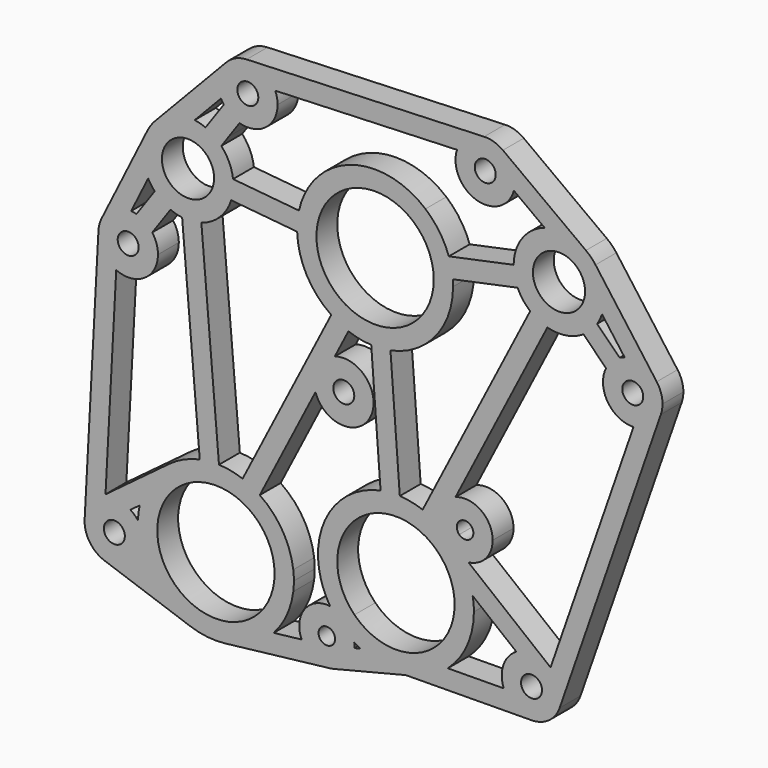
from build123d import *

# Parameters (mm, degrees)
F0_R     = 2.5527
F0_R_2   = 14.2875
F0_R_3   = 6.35
F1_DEPTH = 6.35


# Not quite as in the source:
# - a feature names something its author has since deleted; it is built from what else it names


with BuildPart() as f1:
    # F0 (on Front) → F1 (new body)
    with BuildSketch(Plane.XZ):
        with BuildLine():
            ThreePointArc((10.1027881362, 10.1027881362), (13.1999288208, 5.4675895399), (14.2875, 0))
            ThreePointArc((14.2875, 0), (5.4675895399, -13.1999288208), (-10.1027881362, -10.1027881362))
            Line((-10.1027881362, -10.1027881362), (-12.087424739, -12.087424739))
            ThreePointArc((-12.087424739, -12.087424739), (-10.7962746794, -13.8997241174), (-10.1679167372, -16.0343584679))
            ThreePointArc((-10.1679167372, -16.0343584679), (-9.4333272467, -16.4772424667), (-8.679483979, -16.8864957913))
            ThreePointArc((-8.679483979, -16.8864957913), (-4.3796020882, -18.474476117), (0.1755409055, -18.9856884953))
            ThreePointArc((0.1755409055, -18.9856884953), (2.3991856615, -18.83430621), (4.5897696443, -18.4233872255))
            ThreePointArc((4.5897696443, -18.4233872255), (8.871283082, -16.7865278938), (12.6357418971, -14.1712811333))
            ThreePointArc((12.6357418971, -14.1712811333), (17.326218511, -7.7646206836), (18.9865, 0))
            ThreePointArc((18.9865, 0), (18.9129246484, 1.6698693044), (18.6927688232, 3.3267966532))
            ThreePointArc((18.6927688232, 3.3267966532), (17.6972758772, 6.8770348826), (16.0343584679, 10.1679167372))
            ThreePointArc((16.0343584679, 10.1679167372), (13.8997241174, 10.7962746794), (12.087424739, 12.087424739))
            Line((12.087424739, 12.087424739), (10.1027881362, 10.1027881362))
        make_face()
        with BuildLine():
            ThreePointArc((-10.1027881362, -10.1027881362), (-10.1027881362, 10.1027881362), (10.1027881362, 10.1027881362))
            Line((10.1027881362, 10.1027881362), (12.087424739, 12.087424739))
            ThreePointArc((12.087424739, 12.087424739), (10.7962746794, 13.8997241174), (10.1679167372, 16.0343584679))
            ThreePointArc((10.1679167372, 16.0343584679), (8.3844360103, 17.0349175237), (6.5036895316, 17.8378587484))
            ThreePointArc((6.5036895316, 17.8378587484), (3.7643940626, 18.6095813922), (0.9405215506, 18.9631906984))
            ThreePointArc((0.9405215506, 18.9631906984), (-1.4133229179, 18.933824246), (-3.7454416407, 18.6134050933))
            ThreePointArc((-3.7454416407, 18.6134050933), (-16.2312532017, 9.8505635247), (-18.2403128263, -5.2705))
            Line((-18.2403128263, -5.2705), (-16.1584730714, -5.2705))
            Line((-16.1584730714, -5.2705), (-16.1584730714, -9.9695))
            ThreePointArc((-16.1584730714, -9.9695), (-16.0967214963, -10.0688996082), (-16.0343584679, -10.1679167372))
            ThreePointArc((-16.0343584679, -10.1679167372), (-13.8997241174, -10.7962746794), (-12.087424739, -12.087424739))
            Line((-12.087424739, -12.087424739), (-10.1027881362, -10.1027881362))
        make_face()
        with BuildLine():
            ThreePointArc((10.1679167372, 16.0343584679), (10.7962746794, 13.8997241174), (12.087424739, 12.087424739))
            Line((12.087424739, 12.087424739), (13.425482901, 13.425482901))
            ThreePointArc((13.425482901, 13.425482901), (12.6695294718, 14.1410821797), (11.8754941276, 14.8141763685))
            ThreePointArc((11.8754941276, 14.8141763685), (11.288975975, 15.2658508995), (10.6852962958, 15.6943182496))
            ThreePointArc((10.6852962958, 15.6943182496), (10.4279926298, 15.8664473643), (10.1679167372, 16.0343584679))
        make_face()
        with BuildLine():
            Line((13.425482901, 13.425482901), (12.087424739, 12.087424739))
            ThreePointArc((12.087424739, 12.087424739), (13.8997241174, 10.7962746794), (16.0343584679, 10.1679167372))
            ThreePointArc((16.0343584679, 10.1679167372), (14.8196996494, 11.8686007833), (13.425482901, 13.425482901))
        make_face()
        with BuildLine():
            ThreePointArc((-10.1679167372, -16.0343584679), (-10.7962746794, -13.8997241174), (-12.087424739, -12.087424739))
            Line((-12.087424739, -12.087424739), (-13.425482901, -13.425482901))
            ThreePointArc((-13.425482901, -13.425482901), (-11.8686007833, -14.8196996494), (-10.1679167372, -16.0343584679))
        make_face()
        with BuildLine():
            Line((-13.425482901, -13.425482901), (-12.087424739, -12.087424739))
            ThreePointArc((-12.087424739, -12.087424739), (-13.8997241174, -10.7962746794), (-16.0343584679, -10.1679167372))
            ThreePointArc((-16.0343584679, -10.1679167372), (-14.8196996494, -11.8686007833), (-13.425482901, -13.425482901))
        make_face()
        with BuildLine():
            Line((13.5066179368, 13.5066179368), (13.425482901, 13.425482901))
            ThreePointArc((13.425482901, 13.425482901), (14.8196996494, 11.8686007833), (16.0343584679, 10.1679167372))
            ThreePointArc((16.0343584679, 10.1679167372), (16.8510479224, 10.1196929359), (17.6675435983, 10.1710934346))
            Line((17.6675435983, 10.1710934346), (13.5066179368, 13.5066179368))
        make_face()
        with BuildLine():
            ThreePointArc((11.8754941276, 14.8141763685), (12.6695294718, 14.1410821797), (13.425482901, 13.425482901))
            Line((13.425482901, 13.425482901), (13.5066179368, 13.5066179368))
            Line((13.5066179368, 13.5066179368), (11.8754941276, 14.8141763685))
        make_face()
        with BuildLine():
            ThreePointArc((14.5002054636, 23.1364216251), (11.1025541076, 20.3366145489), (10.1679167372, 16.0343584679))
            ThreePointArc((10.1679167372, 16.0343584679), (10.4279926298, 15.8664473643), (10.6852962958, 15.6943182496))
            Line((10.6852962958, 15.6943182496), (14.5002054636, 23.1364216251))
        make_face()
        with BuildLine():
            ThreePointArc((6.5036895316, 17.8378587484), (8.3844360103, 17.0349175237), (10.1679167372, 16.0343584679))
            ThreePointArc((10.1679167372, 16.0343584679), (11.1025541076, 20.3366145489), (14.5002054636, 23.1364216251))
            Line((14.5002054636, 23.1364216251), (36.8778846589, 66.7906724992))
            ThreePointArc((36.8778846589, 66.7906724992), (34.6718105613, 67.6375732842), (32.6962778947, 68.934212998))
            Line((32.6962778947, 68.934212998), (6.5036895316, 17.8378587484))
        make_face()
        with BuildLine():
            ThreePointArc((17.6675435983, 10.1710934346), (16.8510479224, 10.1196929359), (16.0343584679, 10.1679167372))
            ThreePointArc((16.0343584679, 10.1679167372), (17.6972758772, 6.8770348826), (18.6927688232, 3.3267966532))
            Line((18.6927688232, 3.3267966532), (29.3206645114, -5.1928476183))
            ThreePointArc((29.3206645114, -5.1928476183), (33.5286304822, -4.1961595316), (37.555723844, -5.7718764506))
            Line((37.555723844, -5.7718764506), (17.6675435983, 10.1710934346))
        make_face()
        with BuildLine():
            ThreePointArc((-10.1679167372, -16.0343584679), (-11.8686007833, -14.8196996494), (-13.425482901, -13.425482901))
            ThreePointArc((-13.425482901, -13.425482901), (-14.8196996494, -11.8686007833), (-16.0343584679, -10.1679167372))
            ThreePointArc((-16.0343584679, -10.1679167372), (-22.2468220658, -12.8530103585), (-22.970288636, -19.5821282674))
            ThreePointArc((-22.970288636, -19.5821282674), (-20.1602814757, -22.6773183147), (-16.0638899585, -23.5115354374))
            ThreePointArc((-16.0638899585, -23.5115354374), (-15.6364127746, -23.447956819), (-15.2139078913, -23.3570249376))
            ThreePointArc((-15.2139078913, -23.3570249376), (-11.6731694063, -21.1345234976), (-10.1322290579, -17.2484143236))
            ThreePointArc((-10.1322290579, -17.2484143236), (-10.1228181675, -17.0432931715), (-10.119680227, -16.837980227))
            ThreePointArc((-10.119680227, -16.837980227), (-10.1317501969, -16.4354461624), (-10.1679167372, -16.0343584679))
        make_face()
        with BuildLine():
            ThreePointArc((-14.818680227, -16.837980227), (-18.703570167, -17.610732882), (-15.4101195038, -15.4101195038))
            ThreePointArc((-15.4101195038, -15.4101195038), (-14.972390287, -16.065227572), (-14.818680227, -16.837980227))
        make_face(mode=Mode.SUBTRACT)
        with BuildLine():
            ThreePointArc((10.6852962958, 15.6943182496), (11.288975975, 15.2658508995), (11.8754941276, 14.8141763685))
            Line((11.8754941276, 14.8141763685), (13.5066179368, 13.5066179368))
            Line((13.5066179368, 13.5066179368), (17.6675435983, 10.1710934346))
            ThreePointArc((17.6675435983, 10.1710934346), (21.8732960308, 12.3903797901), (23.556280227, 16.837980227))
            ThreePointArc((23.556280227, 16.837980227), (20.6739731035, 22.3534778058), (14.5002054636, 23.1364216251))
            Line((14.5002054636, 23.1364216251), (10.6852962958, 15.6943182496))
        make_face()
        with BuildLine():
            ThreePointArc((18.857280227, 16.837980227), (17.610732882, 14.972390287), (15.4101195038, 15.4101195038))
            ThreePointArc((15.4101195038, 15.4101195038), (16.065227572, 18.703570167), (18.857280227, 16.837980227))
        make_face(mode=Mode.SUBTRACT)
        with BuildLine():
            ThreePointArc((0.1755409055, -18.9856884953), (-4.3796020882, -18.474476117), (-8.679483979, -16.8864957913))
            Line((-8.679483979, -16.8864957913), (-10.1322290579, -17.2484143236))
            ThreePointArc((-10.1322290579, -17.2484143236), (-11.6731694063, -21.1345234976), (-15.2139078913, -23.3570249376))
            Line((-15.2139078913, -23.3570249376), (2.4158307327, -18.9649748665))
            Line((2.4158307327, -18.9649748665), (0.1755409055, -18.9856884953))
        make_face()
        with BuildLine():
            ThreePointArc((-18.2403128263, -5.2705), (-17.3591263622, -7.6907681145), (-16.1584730714, -9.9695))
            Line((-16.1584730714, -9.9695), (-16.1584730714, -5.2705))
            Line((-16.1584730714, -5.2705), (-18.2403128263, -5.2705))
        make_face()
        with BuildLine():
            ThreePointArc((-16.0638899585, -23.5115354374), (-20.1602814757, -22.6773183147), (-22.970288636, -19.5821282674))
            Line((-22.970288636, -19.5821282674), (-29.7764261148, -20.371597242))
            ThreePointArc((-29.7764261148, -20.371597242), (-35.161229574, -24.5050380312), (-41.6559027226, -26.4800473337))
            Line((-41.6559027226, -26.4800473337), (-16.0638899585, -23.5115354374))
        make_face()
        with BuildLine():
            ThreePointArc((-3.7454416407, 18.6134050933), (-1.4133229179, 18.933824246), (0.9405215506, 18.9631906984))
            Line((0.9405215506, 18.9631906984), (-1.3345583593, 49.4416911273))
            ThreePointArc((-1.3345583593, 49.4416911273), (-3.6666770821, 49.1212719745), (-6.0205215506, 49.0919055222))
            Line((-6.0205215506, 49.0919055222), (-3.7454416407, 18.6134050933))
        make_face()
        with BuildLine():
            ThreePointArc((29.6298751444, 72.9499771349), (30.9304471577, 70.7644612984), (32.6962778947, 68.934212998))
            ThreePointArc((32.6962778947, 68.934212998), (34.6718105613, 67.6375732842), (36.8778846589, 66.7906724992))
            ThreePointArc((36.8778846589, 66.7906724992), (41.4271180616, 66.5549248717), (45.6848221123, 68.1745105325))
            ThreePointArc((45.6848221123, 68.1745105325), (47.5248502349, 69.6571771747), (49.0075168771, 71.4972052973))
            ThreePointArc((49.0075168771, 71.4972052973), (49.6746613221, 72.6923094988), (50.1889265376, 73.9607286137))
            ThreePointArc((50.1889265376, 73.9607286137), (50.617064307, 75.6922004422), (50.7610274096, 77.47))
            ThreePointArc((50.7610274096, 77.47), (50.208206927, 80.9211761095), (48.6050646005, 84.0270031661))
            ThreePointArc((48.6050646005, 84.0270031661), (47.5248502349, 85.2828228253), (46.2690305758, 86.3630371909))
            ThreePointArc((46.2690305758, 86.3630371909), (41.4293864022, 88.3847184614), (36.2027560234, 87.946899128))
            ThreePointArc((36.2027560234, 87.946899128), (32.5255649938, 85.8625656951), (29.9000958465, 82.55))
            ThreePointArc((29.9000958465, 82.55), (28.9861019442, 80.1223430981), (28.6633062214, 77.5484927125))
            ThreePointArc((28.6633062214, 77.5484927125), (28.8993015921, 75.1972568568), (29.6298751444, 72.9499771349))
        make_face()
        with BuildLine():
            ThreePointArc((46.0620274096, 77.47), (36.8722210782, 71.7903873372), (35.9020274096, 82.55))
            ThreePointArc((35.9020274096, 82.55), (42.551833741, 83.1496126628), (46.0620274096, 77.47))
        make_face(mode=Mode.SUBTRACT)
        with BuildLine():
            ThreePointArc((37.555723844, -5.7718764506), (33.5286304822, -4.1961595316), (29.3206645114, -5.1928476183))
            ThreePointArc((29.3206645114, -5.1928476183), (26.1672444912, -9.0578923239), (26.256338269, -14.0453456519))
            ThreePointArc((26.256338269, -14.0453456519), (28.9476060736, -17.4302300454), (33.0870460582, -18.6813900541))
            ThreePointArc((33.0870460582, -18.6813900541), (37.249950733, -17.3202181358), (39.8698682415, -13.8104323061))
            ThreePointArc((39.8698682415, -13.8104323061), (40.170536428, -12.6370549621), (40.2717, -11.43))
            ThreePointArc((40.2717, -11.43), (39.5862059809, -8.352323619), (37.659321687, -5.8565049409))
            ThreePointArc((37.659321687, -5.8565049409), (37.6077179098, -5.8139518102), (37.555723844, -5.7718764506))
        make_face()
        with Locations((33.02, -11.43)):
            Circle(F0_R, mode=Mode.SUBTRACT)
        with BuildLine():
            ThreePointArc((4.5897696443, -18.4233872255), (2.3991856615, -18.83430621), (0.1755409055, -18.9856884953))
            Line((0.1755409055, -18.9856884953), (2.4158307327, -18.9649748665))
            Line((2.4158307327, -18.9649748665), (4.5897696443, -18.4233872255))
        make_face()
        with BuildLine():
            Line((-25.0029803525, -5.2705), (-25.0029803525, -9.9695))
            ThreePointArc((-25.0029803525, -9.9695), (-24.893567057, -8.7970138243), (-24.8570491337, -7.62))
            ThreePointArc((-24.8570491337, -7.62), (-24.893567057, -6.4429861757), (-25.0029803525, -5.2705))
        make_face()
        with BuildLine():
            ThreePointArc((-29.7764261148, -20.371597242), (-26.5872473381, -15.5387897174), (-25.0029803525, -9.9695))
            Line((-25.0029803525, -9.9695), (-25.0029803525, -5.2705))
            ThreePointArc((-25.0029803525, -5.2705), (-27.6442418047, 2.283010871), (-33.1629165809, 8.0774924915))
            ThreePointArc((-33.1629165809, 8.0774924915), (-35.1875075447, 9.2785243811), (-37.3451600732, 10.2197904099))
            ThreePointArc((-37.3451600732, 10.2197904099), (-40.1777850684, 11.0092607494), (-43.0983409674, 11.3518698878))
            ThreePointArc((-43.0983409674, 11.3518698878), (-45.4517582606, 11.298267512), (-47.7804539971, 10.9538515754))
            ThreePointArc((-47.7804539971, 10.9538515754), (-51.6694427495, 9.6786291759), (-55.1947929153, 7.5996073162))
            ThreePointArc((-55.1947929153, 7.5996073162), (-59.8231534442, 2.6337519149), (-62.4088249945, -3.642850963))
            ThreePointArc((-62.4088249945, -3.642850963), (-62.6907023453, -5.3239167985), (-62.8206763208, -7.0234884945))
            ThreePointArc((-62.8206763208, -7.0234884945), (-61.7115198037, -9.1038158537), (-61.3283, -11.43))
            ThreePointArc((-61.3283, -11.43), (-61.4374580323, -12.6834939688), (-61.761645872, -13.8992508732))
            ThreePointArc((-61.761645872, -13.8992508732), (-61.1262796106, -15.4809420245), (-60.3516188327, -16.9992759349))
            ThreePointArc((-60.3516188327, -16.9992759349), (-55.997100169, -22.2069249495), (-50.088980786, -25.5499125967))
            ThreePointArc((-50.088980786, -25.5499125967), (-45.925061306, -26.492055779), (-41.6559027226, -26.4800473337))
            ThreePointArc((-41.6559027226, -26.4800473337), (-35.161229574, -24.5050380312), (-29.7764261148, -20.371597242))
        make_face()
        with Locations((-43.8435491337, -7.62)):
            Circle(F0_R_2, mode=Mode.SUBTRACT)
        with BuildLine():
            ThreePointArc((-6.0205215506, 49.0919055222), (-3.6666770821, 49.1212719745), (-1.3345583593, 49.4416911273))
            ThreePointArc((-1.3345583593, 49.4416911273), (9.6101329123, 56.026497912), (13.9065, 68.0550962206))
            ThreePointArc((13.9065, 68.0550962206), (13.8901085456, 68.8438699637), (13.8409624846, 69.6312817761))
            ThreePointArc((13.8409624846, 69.6312817761), (13.5004886175, 71.9605571391), (12.8743935617, 74.2297973537))
            ThreePointArc((12.8743935617, 74.2297973537), (10.5910398053, 78.7745035583), (7.1831540264, 82.55))
            Line((7.1831540264, 82.55), (-17.3431540264, 82.55))
            ThreePointArc((-17.3431540264, 82.55), (-21.3280411608, 77.8779441115), (-23.6133618959, 72.1784054603))
            ThreePointArc((-23.6133618959, 72.1784054603), (-23.9811558005, 69.8532874387), (-24.0583991873, 67.5005274361))
            ThreePointArc((-24.0583991873, 67.5005274361), (-21.7305728292, 58.9311931791), (-15.7606325528, 52.357603729))
            ThreePointArc((-15.7606325528, 52.357603729), (-13.736041589, 51.1565718394), (-11.5783890605, 50.2153058107))
            ThreePointArc((-11.5783890605, 50.2153058107), (-8.8416292776, 49.4449557744), (-6.0205215506, 49.0919055222))
        make_face()
        with Locations((-5.08, 68.0550962206)):
            Circle(F0_R_2, mode=Mode.SUBTRACT)
        with BuildLine():
            Line((13.8409624846, 69.6312817761), (29.6298751444, 72.9499771349))
            ThreePointArc((29.6298751444, 72.9499771349), (28.8993015921, 75.1972568568), (28.6633062214, 77.5484927125))
            Line((28.6633062214, 77.5484927125), (12.8743935617, 74.2297973537))
            ThreePointArc((12.8743935617, 74.2297973537), (13.5004886175, 71.9605571391), (13.8409624846, 69.6312817761))
        make_face()
        with BuildLine():
            ThreePointArc((49.0075168771, 71.4972052973), (47.5248502349, 69.6571771747), (45.6848221123, 68.1745105325))
            Line((45.6848221123, 68.1745105325), (51.1600582452, 62.6992743996))
            ThreePointArc((51.1600582452, 62.6992743996), (52.5448134066, 64.637214003), (54.48275301, 66.0219691644))
            Line((54.48275301, 66.0219691644), (49.0075168771, 71.4972052973))
        make_face()
        with BuildLine():
            Line((26.256338269, -14.0453456519), (12.6357418971, -14.1712811333))
            ThreePointArc((12.6357418971, -14.1712811333), (8.871283082, -16.7865278938), (4.5897696443, -18.4233872255))
            Line((4.5897696443, -18.4233872255), (2.4158307327, -18.9649748665))
            Line((2.4158307327, -18.9649748665), (33.0870460582, -18.6813900541))
            ThreePointArc((33.0870460582, -18.6813900541), (28.9476060736, -17.4302300454), (26.256338269, -14.0453456519))
        make_face()
        with BuildLine():
            Line((57.855717147, 52.2601016531), (37.659321687, -5.8565049409))
            ThreePointArc((37.659321687, -5.8565049409), (39.5862059809, -8.352323619), (40.2717, -11.43))
            ThreePointArc((40.2717, -11.43), (40.170536428, -12.6370549621), (39.8698682415, -13.8104323061))
            Line((39.8698682415, -13.8104323061), (64.5224078933, 57.1290554518))
            ThreePointArc((64.5224078933, 57.1290554518), (61.9495258403, 53.6533335563), (57.855717147, 52.2601016531))
        make_face()
        with BuildLine():
            ThreePointArc((54.48275301, 66.0219691644), (52.5448134066, 64.637214003), (51.1600582452, 62.6992743996))
            ThreePointArc((51.1600582452, 62.6992743996), (51.5685160683, 55.5943825253), (57.855717147, 52.2601016531))
            ThreePointArc((57.855717147, 52.2601016531), (61.9495258403, 53.6533335563), (64.5224078933, 57.1290554518))
            ThreePointArc((64.5224078933, 57.1290554518), (64.8230760798, 58.3024327958), (64.9242396518, 59.5094877579))
            ThreePointArc((64.9242396518, 59.5094877579), (64.5614114959, 61.774570009), (63.5092341759, 63.8129921347))
            ThreePointArc((63.5092341759, 63.8129921347), (60.0218780259, 66.3700826369), (55.6990804779, 66.4874969137))
            ThreePointArc((55.6990804779, 66.4874969137), (55.0804447732, 66.2820941269), (54.48275301, 66.0219691644))
        make_face()
        with Locations((57.6725396518, 59.5094877579)):
            Circle(F0_R, mode=Mode.SUBTRACT)
        with BuildLine():
            ThreePointArc((-37.3451600732, 10.2197904099), (-35.1875075447, 9.2785243811), (-33.1629165809, 8.0774924915))
            Line((-33.1629165809, 8.0774924915), (-19.5912999954, 34.5723159514))
            ThreePointArc((-19.5912999954, 34.5723159514), (-19.1542190111, 40.1360867875), (-14.8944004468, 43.7417117684))
            Line((-14.8944004468, 43.7417117684), (-11.5783890605, 50.2153058107))
            ThreePointArc((-11.5783890605, 50.2153058107), (-13.736041589, 51.1565718394), (-15.7606325528, 52.357603729))
            Line((-15.7606325528, 52.357603729), (-37.3451600732, 10.2197904099))
        make_face()
        with BuildLine():
            Line((-70.965378912, -18.2781472192), (-50.088980786, -25.5499125967))
            ThreePointArc((-50.088980786, -25.5499125967), (-55.997100169, -22.2069249495), (-60.3516188327, -16.9992759349))
            Line((-60.3516188327, -16.9992759349), (-63.0098570833, -16.0733458602))
            ThreePointArc((-63.0098570833, -16.0733458602), (-66.6432584841, -18.4182891462), (-70.965378912, -18.2781472192))
        make_face()
        with BuildLine():
            ThreePointArc((50.7610274096, 77.47), (50.617064307, 75.6922004422), (50.1889265376, 73.9607286137))
            Line((50.1889265376, 73.9607286137), (55.6990804779, 66.4874969137))
            ThreePointArc((55.6990804779, 66.4874969137), (60.0218780259, 66.3700826369), (63.5092341759, 63.8129921347))
            Line((63.5092341759, 63.8129921347), (48.6050646005, 84.0270031661))
            ThreePointArc((48.6050646005, 84.0270031661), (50.208206927, 80.9211761095), (50.7610274096, 77.47))
        make_face()
        with BuildLine():
            ThreePointArc((-14.8944004468, 43.7417117684), (-19.1542190111, 40.1360867875), (-19.5912999954, 34.5723159514))
            Line((-19.5912999954, 34.5723159514), (-14.8944004468, 43.7417117684))
        make_face()
        with BuildLine():
            Line((-14.8944004468, 43.7417117684), (-19.5912999954, 34.5723159514))
            ThreePointArc((-19.5912999954, 34.5723159514), (-11.5568655562, 29.6689667971), (-5.4483, 36.83))
            ThreePointArc((-5.4483, 36.83), (-8.4178265349, 42.6823621987), (-14.8944004468, 43.7417117684))
        make_face()
        with Locations((-12.7, 36.83)):
            Circle(F0_R, mode=Mode.SUBTRACT)
        with BuildLine():
            Line((-63.0098570833, -16.0733458602), (-60.3516188327, -16.9992759349))
            ThreePointArc((-60.3516188327, -16.9992759349), (-61.1262796106, -15.4809420245), (-61.761645872, -13.8992508732))
            ThreePointArc((-61.761645872, -13.8992508732), (-62.2910901573, -15.0406461859), (-63.0098570833, -16.0733458602))
        make_face()
        with BuildLine():
            ThreePointArc((-75.8213755396, -11.0431755126), (-74.6011962447, -15.4713300624), (-70.965378912, -18.2781472192))
            ThreePointArc((-70.965378912, -18.2781472192), (-66.6432584841, -18.4182891462), (-63.0098570833, -16.0733458602))
            ThreePointArc((-63.0098570833, -16.0733458602), (-62.2910901573, -15.0406461859), (-61.761645872, -13.8992508732))
            ThreePointArc((-61.761645872, -13.8992508732), (-62.6087673365, -10.5102885761), (-62.8206763208, -7.0234884945))
            ThreePointArc((-62.8206763208, -7.0234884945), (-63.6690383747, -6.0943080294), (-64.6652410316, -5.3257543374))
            ThreePointArc((-64.6652410316, -5.3257543374), (-67.625936904, -4.2413341642), (-70.7669999633, -4.5159430108))
            ThreePointArc((-70.7669999633, -4.5159430108), (-71.8873888003, -4.9764480932), (-72.9154917721, -5.6170262357))
            ThreePointArc((-72.9154917721, -5.6170262357), (-74.9727097683, -8.0064908781), (-75.8213755396, -11.0431755126))
        make_face()
        with Locations((-68.58, -11.43)):
            Circle(F0_R, mode=Mode.SUBTRACT)
        with BuildLine():
            Line((-17.3431540264, 82.55), (7.1831540264, 82.55))
            ThreePointArc((7.1831540264, 82.55), (-5.08, 87.0415962206), (-17.3431540264, 82.55))
        make_face()
        with BuildLine():
            Line((28.7295243233, 93.4570530682), (36.2027560234, 87.946899128))
            ThreePointArc((36.2027560234, 87.946899128), (41.4293864022, 88.3847184614), (46.2690305758, 86.3630371909))
            Line((46.2690305758, 86.3630371909), (26.0550195443, 101.2672067663))
            ThreePointArc((26.0550195443, 101.2672067663), (28.224338183, 98.7000252181), (29.0032151675, 95.4305122421))
            ThreePointArc((29.0032151675, 95.4305122421), (28.9344665764, 94.434338589), (28.7295243233, 93.4570530682))
        make_face()
        with BuildLine():
            ThreePointArc((-47.7804539971, 10.9538515754), (-45.4517582606, 11.298267512), (-43.0983409674, 11.3518698878))
            Line((-43.0983409674, 11.3518698878), (-47.3895269006, 61.8315009716))
            ThreePointArc((-47.3895269006, 61.8315009716), (-49.7091796418, 61.3807072004), (-52.0716399303, 61.4334826592))
            Line((-52.0716399303, 61.4334826592), (-47.7804539971, 10.9538515754))
        make_face()
        with BuildLine():
            ThreePointArc((-62.8206763208, -7.0234884945), (-62.6087673365, -10.5102885761), (-61.761645872, -13.8992508732))
            ThreePointArc((-61.761645872, -13.8992508732), (-61.4374580323, -12.6834939688), (-61.3283, -11.43))
            ThreePointArc((-61.3283, -11.43), (-61.7115198037, -9.1038158537), (-62.8206763208, -7.0234884945))
        make_face()
        with BuildLine():
            Line((-72.4552775613, 51.9703625624), (-75.8213755396, -11.0431755126))
            ThreePointArc((-75.8213755396, -11.0431755126), (-74.9727097683, -8.0064908781), (-72.9154917721, -5.6170262357))
            Line((-72.9154917721, -5.6170262357), (-70.7391085237, -3.9938137374))
            Line((-70.7391085237, -3.9938137374), (-68.125033349, 44.9418163641))
            ThreePointArc((-68.125033349, 44.9418163641), (-71.387917274, 47.7797651384), (-72.4552775613, 51.9703625624))
        make_face()
        with BuildLine():
            Line((-40.1198012444, 69.0285542105), (-24.0583991873, 67.5005274361))
            ThreePointArc((-24.0583991873, 67.5005274361), (-23.9811558005, 69.8532874387), (-23.6133618959, 72.1784054603))
            Line((-23.6133618959, 72.1784054603), (-39.674763953, 73.7064322347))
            ThreePointArc((-39.674763953, 73.7064322347), (-39.6157539425, 73.0493913967), (-39.5960605383, 72.39))
            ThreePointArc((-39.5960605383, 72.39), (-39.7277808648, 70.6889986682), (-40.1198012444, 69.0285542105))
        make_face()
        with BuildLine():
            ThreePointArc((14.8704771454, 97.719282355), (19.6198490413, 88.4991954541), (28.7295243233, 93.4570530682))
            ThreePointArc((28.7295243233, 93.4570530682), (28.9344665764, 94.434338589), (29.0032151675, 95.4305122421))
            ThreePointArc((29.0032151675, 95.4305122421), (28.224338183, 98.7000252181), (26.0550195443, 101.2672067663))
            ThreePointArc((26.0550195443, 101.2672067663), (23.8831812936, 102.3618290302), (21.4715701429, 102.6768067209))
            ThreePointArc((21.4715701429, 102.6768067209), (17.3967268249, 101.229044072), (14.8704771454, 97.719282355))
        make_face()
        with Locations((21.7515151675, 95.4305122421)):
            Circle(F0_R, mode=Mode.SUBTRACT)
        with BuildLine():
            ThreePointArc((-52.0716399303, 61.4334826592), (-49.7091796418, 61.3807072004), (-47.3895269006, 61.8315009716))
            ThreePointArc((-47.3895269006, 61.8315009716), (-42.8715827267, 64.5380293103), (-40.1198012444, 69.0285542105))
            ThreePointArc((-40.1198012444, 69.0285542105), (-39.7277808648, 70.6889986682), (-39.5960605383, 72.39))
            ThreePointArc((-39.5960605383, 72.39), (-39.6157539425, 73.0493913967), (-39.674763953, 73.7064322347))
            ThreePointArc((-39.674763953, 73.7064322347), (-40.6136295887, 77.0215002001), (-42.5279553584, 79.8861993369))
            ThreePointArc((-42.5279553584, 79.8861993369), (-44.2746130083, 81.4176131545), (-46.302849005, 82.55))
            Line((-46.302849005, 82.55), (-54.9872720717, 82.55))
            ThreePointArc((-54.9872720717, 82.55), (-56.9463680029, 81.4660082215), (-58.646707795, 80.0093203227))
            ThreePointArc((-58.646707795, 80.0093203227), (-59.6958714757, 78.7274460452), (-60.5416041625, 77.3031278524))
            ThreePointArc((-60.5416041625, 77.3031278524), (-61.6921761605, 72.1859474801), (-60.3534134459, 67.1147478902))
            ThreePointArc((-60.3534134459, 67.1147478902), (-59.6267024068, 65.9549001293), (-58.7621657183, 64.8938006631))
            ThreePointArc((-58.7621657183, 64.8938006631), (-56.9825065836, 63.3391890627), (-54.9129702621, 62.1985649887))
            ThreePointArc((-54.9129702621, 62.1985649887), (-53.5178882942, 61.7210140273), (-52.0716399303, 61.4334826592))
        make_face()
        with Locations((-50.6450605383, 72.39)):
            Circle(F0_R_3, mode=Mode.SUBTRACT)
        with BuildLine():
            Line((-70.7391085237, -3.9938137374), (-72.9154917721, -5.6170262357))
            ThreePointArc((-72.9154917721, -5.6170262357), (-71.8873888003, -4.9764480932), (-70.7669999633, -4.5159430108))
            Line((-70.7669999633, -4.5159430108), (-70.7391085237, -3.9938137374))
        make_face()
        with BuildLine():
            ThreePointArc((-71.7092197336, 54.8081311828), (-72.2272762494, 53.4273750614), (-72.4552775613, 51.9703625624))
            ThreePointArc((-72.4552775613, 51.9703625624), (-71.387917274, 47.7797651384), (-68.125033349, 44.9418163641))
            ThreePointArc((-68.125033349, 44.9418163641), (-61.2467555759, 45.5132084326), (-57.9622020217, 51.5835380751))
            ThreePointArc((-57.9622020217, 51.5835380751), (-58.3189939198, 53.8301789356), (-59.3542604787, 55.8557452186))
            ThreePointArc((-59.3542604787, 55.8557452186), (-61.0544977782, 57.5237829546), (-63.2034559348, 58.550980893))
            ThreePointArc((-63.2034559348, 58.550980893), (-63.8372376428, 58.7033658874), (-64.4821427006, 58.7982231816))
            ThreePointArc((-64.4821427006, 58.7982231816), (-68.7188784654, 57.9319467748), (-71.7092197336, 54.8081311828))
        make_face()
        with Locations((-65.2139020217, 51.5835380751)):
            Circle(F0_R, mode=Mode.SUBTRACT)
        with BuildLine():
            Line((-42.5279553584, 79.8861993369), (-40.6627420538, 82.55))
            Line((-40.6627420538, 82.55), (-46.302849005, 82.55))
            ThreePointArc((-46.302849005, 82.55), (-44.2746130083, 81.4176131545), (-42.5279553584, 79.8861993369))
        make_face()
        with BuildLine():
            Line((-46.302849005, 82.55), (-40.6627420538, 82.55))
            Line((-40.6627420538, 82.55), (-38.0866651419, 86.229019107))
            ThreePointArc((-38.0866651419, 86.229019107), (-40.2356232985, 87.2562170454), (-41.935860598, 88.9242547814))
            Line((-41.935860598, 88.9242547814), (-46.3771508146, 82.5814350113))
            ThreePointArc((-46.3771508146, 82.5814350113), (-46.3399712181, 82.5657853232), (-46.302849005, 82.55))
        make_face()
        with BuildLine():
            Line((-29.3922701747, 96.0092861737), (14.8704771454, 97.719282355))
            ThreePointArc((14.8704771454, 97.719282355), (17.3967268249, 101.229044072), (21.4715701429, 102.6768067209))
            Line((21.4715701429, 102.6768067209), (-36.3561640796, 100.4427564037))
            ThreePointArc((-36.3561640796, 100.4427564037), (-32.1817703243, 99.3136853125), (-29.3922701747, 96.0092861737))
        make_face()
        with BuildLine():
            ThreePointArc((-62.4088249945, -3.642850963), (-59.8231534442, 2.6337519149), (-55.1947929153, 7.5996073162))
            Line((-55.1947929153, 7.5996073162), (-70.7391085237, -3.9938137374))
            Line((-70.7391085237, -3.9938137374), (-70.7669999633, -4.5159430108))
            ThreePointArc((-70.7669999633, -4.5159430108), (-67.625936904, -4.2413341642), (-64.6652410316, -5.3257543374))
            Line((-64.6652410316, -5.3257543374), (-62.4088249945, -3.642850963))
        make_face()
        with BuildLine():
            Line((-60.5416041625, 77.3031278524), (-71.7092197336, 54.8081311828))
            ThreePointArc((-71.7092197336, 54.8081311828), (-68.7188784654, 57.9319467748), (-64.4821427006, 58.7982231816))
            Line((-64.4821427006, 58.7982231816), (-60.3534134459, 67.1147478902))
            ThreePointArc((-60.3534134459, 67.1147478902), (-61.6921761605, 72.1859474801), (-60.5416041625, 77.3031278524))
        make_face()
        with BuildLine():
            Line((-54.9872720717, 82.55), (-46.302849005, 82.55))
            ThreePointArc((-46.302849005, 82.55), (-46.3399712181, 82.5657853232), (-46.3771508146, 82.5814350113))
            ThreePointArc((-46.3771508146, 82.5814350113), (-47.669947115, 83.0309163665), (-49.0083973109, 83.3171100699))
            ThreePointArc((-49.0083973109, 83.3171100699), (-52.0511588186, 83.3491645953), (-54.9872720717, 82.55))
        make_face()
        with BuildLine():
            ThreePointArc((-41.935860598, 88.9242547814), (-40.2356232985, 87.2562170454), (-38.0866651419, 86.229019107))
            ThreePointArc((-38.0866651419, 86.229019107), (-31.7168612467, 87.4013646532), (-28.824519055, 93.1964619249))
            ThreePointArc((-28.824519055, 93.1964619249), (-28.9678737839, 94.631237307), (-29.3922701747, 96.0092861737))
            ThreePointArc((-29.3922701747, 96.0092861737), (-32.1817703243, 99.3136853125), (-36.3561640796, 100.4427564037))
            ThreePointArc((-36.3561640796, 100.4427564037), (-39.0612309681, 99.8053087811), (-41.3278748982, 98.1971882517))
            ThreePointArc((-41.3278748982, 98.1971882517), (-43.2405444095, 94.3187787718), (-42.605528983, 90.0412654566))
            ThreePointArc((-42.605528983, 90.0412654566), (-42.2958217634, 89.4676960379), (-41.935860598, 88.9242547814))
        make_face()
        with Locations((-36.076219055, 93.1964619249)):
            Circle(F0_R, mode=Mode.SUBTRACT)
        with BuildLine():
            Line((-59.3542604787, 55.8557452186), (-54.9129702621, 62.1985649887))
            ThreePointArc((-54.9129702621, 62.1985649887), (-56.9825065836, 63.3391890627), (-58.7621657183, 64.8938006631))
            Line((-58.7621657183, 64.8938006631), (-63.2034559348, 58.550980893))
            ThreePointArc((-63.2034559348, 58.550980893), (-61.0544977782, 57.5237829546), (-59.3542604787, 55.8557452186))
        make_face()
        with BuildLine():
            ThreePointArc((-58.646707795, 80.0093203227), (-56.9463680029, 81.4660082215), (-54.9872720717, 82.55))
            Line((-54.9872720717, 82.55), (-56.2274244053, 82.55))
            Line((-56.2274244053, 82.55), (-58.646707795, 80.0093203227))
        make_face()
        with BuildLine():
            Line((-56.2274244053, 82.55), (-54.9872720717, 82.55))
            ThreePointArc((-54.9872720717, 82.55), (-52.0511588186, 83.3491645953), (-49.0083973109, 83.3171100699))
            Line((-49.0083973109, 83.3171100699), (-42.605528983, 90.0412654566))
            ThreePointArc((-42.605528983, 90.0412654566), (-43.2405444095, 94.3187787718), (-41.3278748982, 98.1971882517))
            Line((-41.3278748982, 98.1971882517), (-56.2274244053, 82.55))
        make_face()
    extrude(amount=F1_DEPTH)


solid = f1.part
